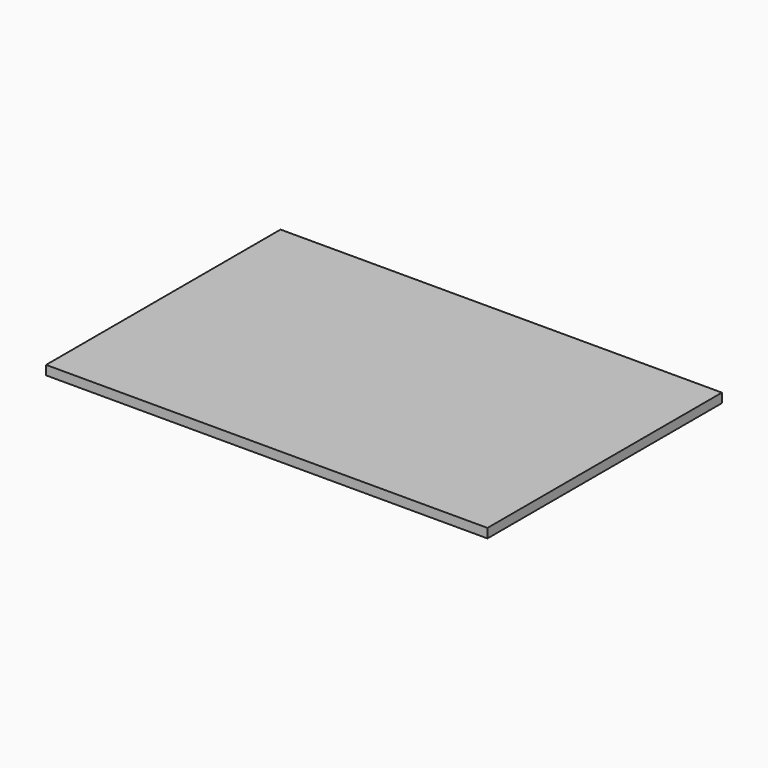
from build123d import *

# Parameters (mm, degrees)
F0_W     = 755.65
F0_H     = 501.65
F1_DEPTH = 15.875


# Not quite as in the source:
# - a length typed as a fraction of an inch, garbled in the dataset ("3 / 203.2 mm" for 3/8 in), is restored


with BuildPart() as f1:
    # F0 (on Top) → F1 (new body)
    with BuildSketch(Plane.XY):
        with Locations((377.825, 250.825)):
            Rectangle(F0_W, F0_H)
    extrude(amount=F1_DEPTH)


solid = f1.part
